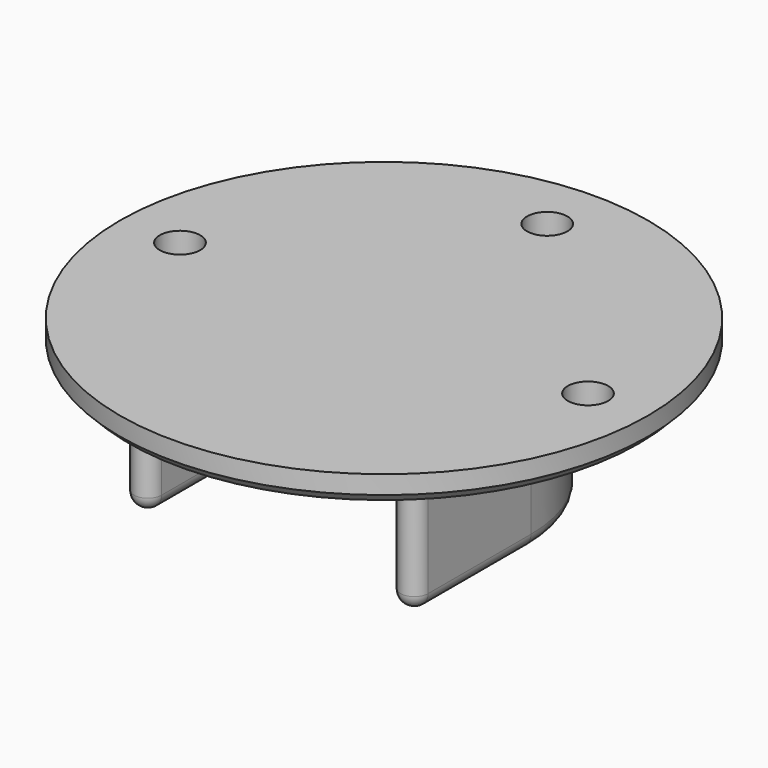
from build123d import *

# Parameters (mm, degrees)
F0_R     = 36.5
F0_R_2   = 2.794
F1_DEPTH = 3.81
F2_SIZE  = 1.27
F4_DEPTH = 17.78
F5_R     = 1.90499


# Not quite as in the source:
# - a fillet or chamfer is up to 0.001 mm smaller than in the source, because OpenCascade refuses the exact size


with BuildPart() as f1:
    # F0 (on Top) → F1 (new body)
    with BuildSketch(Plane.XY):
        Circle(F0_R)
        with Locations((-28.194, 0)):
            Circle(F0_R_2, mode=Mode.SUBTRACT)
        with Locations((28.194, 0)):
            Circle(F0_R_2, mode=Mode.SUBTRACT)
        with Locations((0, 28.194)):
            Circle(F0_R_2, mode=Mode.SUBTRACT)
    extrude(amount=F1_DEPTH)

    # F2
    f2_edges = [f1.edges().sort_by_distance(p)[0] for p in [
        (-36.5, 0, 0),
    ]]
    chamfer(f2_edges, length=F2_SIZE)

    # F3 (on face) → F4 (join)
    with BuildSketch(Plane(origin=(0, 0, 0), x_dir=(1, 0, 0), z_dir=(0, 0, -1))):
        with BuildLine():
            Line((16.51, 17.78), (16.51, 0))
            ThreePointArc((16.51, 0), (0, -16.51), (-16.51, 0))
            Line((-16.51, 0), (-16.51, 17.78))
            ThreePointArc((-16.51, 17.78), (-18.415, 19.685), (-20.32, 17.78))
            Line((-20.32, 17.78), (-20.32, 0))
            ThreePointArc((-20.32, 0), (0, -20.32), (20.32, 0))
            Line((20.32, 0), (20.32, 17.78))
            ThreePointArc((20.32, 17.78), (18.415, 19.685), (16.51, 17.78))
        make_face()
    extrude(amount=F4_DEPTH)

    # F5 (radius 1.905 in the source; OpenCascade refuses exactly that, so slightly less here)
    f5_edges = [f1.edges().sort_by_distance(p)[0] for p in [
        (-20.32, -8.89, -17.78),
        (-16.51, -8.89, -17.78),
        (-18.415, -19.685, -17.78),
        (0, 20.32, -17.78),
        (0, 16.51, -17.78),
        (16.51, -8.89, -17.78),
        (20.32, -8.89, -17.78),
        (18.415, -19.685, -17.78),
    ]]
    fillet(f5_edges, radius=F5_R)


solid = f1.part
